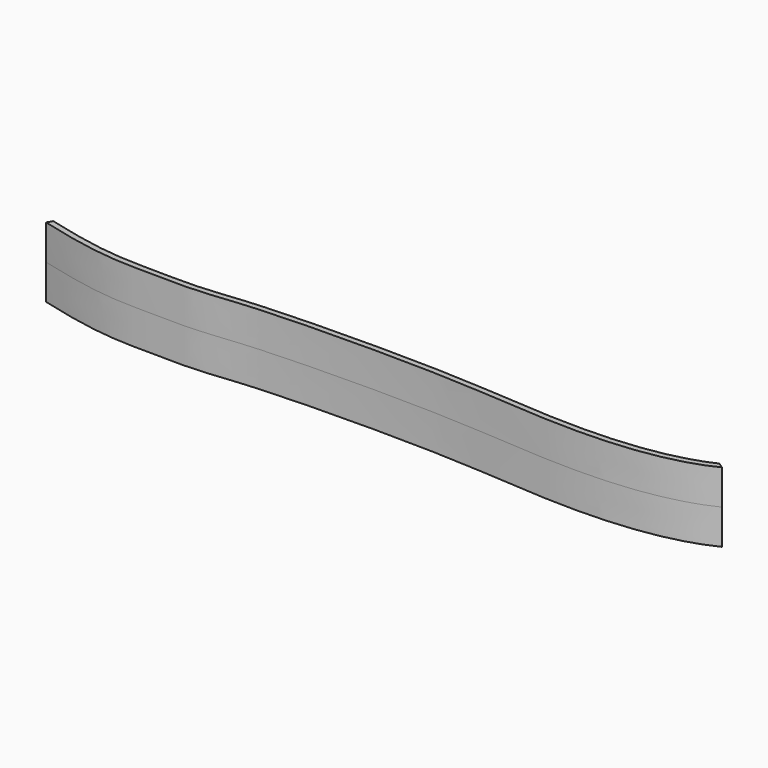
from build123d import *

# Parameters (mm, degrees)
F1_DEPTH = 76.2


# Not quite as in the source:
# - ends of sketch curves that miss each other by under 0.0002 mm in the source are joined
# - the dataset's text gives a spline's control points without its knots; the knots are read off the source's solid


with BuildPart() as f1:
    # F0 (on Top) → F1 (new body, symmetric)
    with BuildSketch(Plane.XY):
        with BuildLine():
            Line((-343.7498003572, 47.0541436232), (-350.2753078938, 35.6421843171))
            add(Edge.make_bspline(
                [(-350.2753078938, 35.6421843171), (-215.7750274511, 0), (-130.7092147924, 1.2778233236), (6.9112403788, -3.0173373582), (128.1929020364, 16.5167814462), (557.9135287963, 21.395786858), (790.9149290877, -8.114036742), (1023.3768942921, 5.47974739), (1111.2263998195, 49.2291151305)],
                knots=[0, 0, 0, 0, 0.1701471791, 0.2847863071, 0.4077713836, 0.6304881518, 0.80765018, 1, 1, 1, 1], degree=3))
            Line((1111.2263998195, 49.2291151305), (1099.320736712, 57.5787103522))
            add(Edge.make_bspline(
                [(-343.7498003572, 47.0541436232), (-320.533596793, 40.9424641987), (-278.2851639822, 30.7135477964), (-236.3068382895, 22.6414623427), (-207.3892895573, 18.3286915423), (-187.9155193381, 16.044387482), (-170.2237251852, 14.530809674), (-153.8708032362, 13.6111257692), (-140.9854038197, 13.1953517076), (-130.9005982957, 12.9875736598), (-123.3949398693, 12.8727203986), (-117.1440223506, 12.7930585564), (-112.1208009891, 12.7281401069), (-107.0711163989, 12.6582520415), (-100.7365905068, 12.5593404952), (-93.1102975594, 12.430109505), (-85.4700928308, 12.2969781967), (-75.2794113908, 12.1235366485), (-62.5619315234, 11.9314474572), (-47.4250979102, 11.795042318), (-32.5043462199, 11.8064798239), (-17.895211509, 12.0197815809), (-3.688660886, 12.4843413455), (9.9968147251, 13.2615337206), (23.5780544567, 14.323487163), (37.4259745282, 15.6103304358), (56.7292814437, 17.553564258), (77.9901983572, 19.719331655), (102.5698463947, 21.8592748109), (123.0018854391, 23.3901419384), (145.7830872514, 24.7814003549), (178.9407271515, 26.4368656484), (224.9417690306, 28.1260434413), (285.263145192, 29.5047643312), (348.5172361779, 30.1938880969), (401.8453240504, 30.1579571774), (443.7810778046, 29.7414455679), (474.595879308, 29.2296587643), (499.5165252968, 28.6323674449), (518.861809931, 28.0491280233), (533.0417814749, 27.5583825428), (546.8570468749, 27.0130339185), (560.2806627619, 26.4145530699), (573.3449265232, 25.769962789), (590.3187659051, 24.8571165661), (610.7694468865, 23.6317634679), (634.2985788494, 22.0766853401), (657.0318724851, 20.4871482642), (679.1862893619, 18.9130762234), (700.9805765097, 17.4039813469), (722.6356329888, 16.0088745709), (744.3746060492, 14.7763036929), (762.7481063881, 13.9247910545), (777.7147948873, 13.3730459493), (789.1025751995, 13.029964793), (800.6801183683, 12.7637985112), (812.4814466338, 12.5800740555), (824.4968234003, 12.4881649994), (840.7677003173, 12.5033038945), (861.5201790506, 12.8077494117), (886.8996615613, 13.7179888512), (921.1263782889, 15.7745294615), (964.1691065023, 20.1426520399), (1014.728600317, 28.9384153923), (1060.2687181222, 41.2802951653), (1087.4724653391, 52.0190924189), (1099.320736712, 57.5787103522)],
                knots=[0.0013954181, 0.0013954181, 0.0013954181, 0.0013954181, 0.03125, 0.0625, 0.078125, 0.09375, 0.109375, 0.125, 0.140625, 0.1484375, 0.15625, 0.1640625, 0.16796875, 0.171875, 0.1796875, 0.1875, 0.1953125, 0.203125, 0.21875, 0.234375, 0.25, 0.265625, 0.28125, 0.296875, 0.3125, 0.328125, 0.34375, 0.375, 0.390625, 0.40625, 0.421875, 0.4375, 0.46875, 0.5, 0.53125, 0.5625, 0.578125, 0.59375, 0.609375, 0.6171875, 0.625, 0.6328125, 0.640625, 0.6484375, 0.65625, 0.671875, 0.6875, 0.703125, 0.71875, 0.734375, 0.75, 0.765625, 0.78125, 0.7890625, 0.796875, 0.8046875, 0.8125, 0.8203125, 0.828125, 0.84375, 0.859375, 0.875, 0.90625, 0.9375, 0.96875, 0.9952912854, 0.9952912854, 0.9952912854, 0.9952912854], degree=3))
        make_face()
    extrude(amount=F1_DEPTH, both=True)


solid = f1.part
